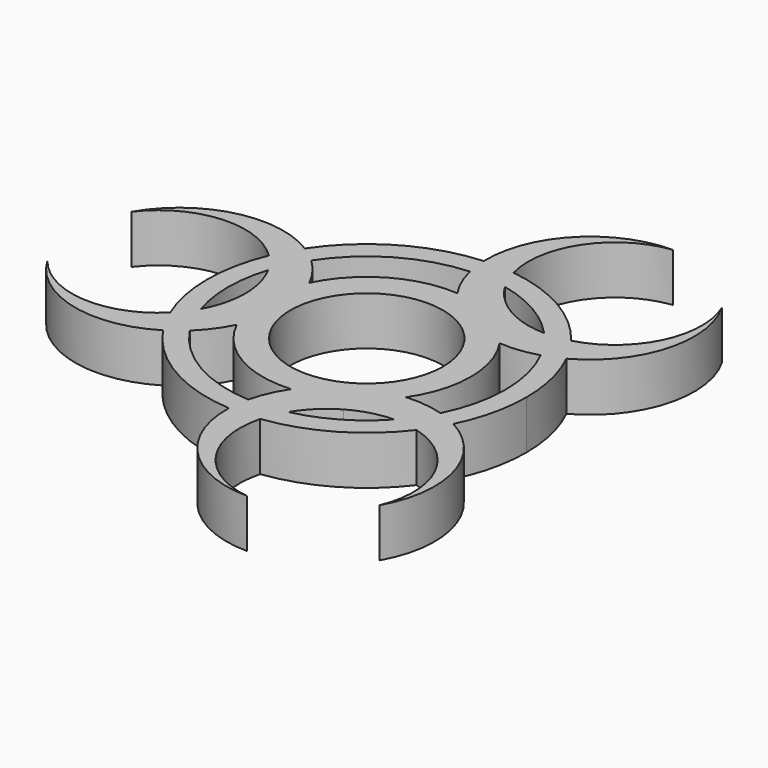
from build123d import *

# Parameters (mm, degrees)
F0_R     = 11
F1_DEPTH = 7
F2_COUNT = 3


# Not quite as in the source:
# - a feature names something its author has since deleted; it is built from what else it names


with BuildPart() as f1:
    # F0 (on Top) → F1 (new body)
    with BuildSketch(Plane.XY):
        with BuildLine():
            ThreePointArc((-13.5, -6.5383484153), (3.3541019662, -14.6201915172), (15, 0))
            ThreePointArc((15, 0), (3.3541019662, 14.6201915172), (-13.5, 6.5383484153))
            ThreePointArc((-13.5, 6.5383484153), (-12.3798084828, 3.3541019662), (-12, 0))
            ThreePointArc((-12, 0), (-12.3798084828, -3.3541019662), (-13.5, -6.5383484153))
        make_face()
        Circle(F0_R, mode=Mode.SUBTRACT)
        with BuildLine():
            ThreePointArc((-12, 0), (-12.3798084828, 3.3541019662), (-13.5, 6.5383484153))
            ThreePointArc((-13.5, 6.5383484153), (-15, 0), (-13.5, -6.5383484153))
            ThreePointArc((-13.5, -6.5383484153), (-12.3798084828, -3.3541019662), (-12, 0))
        make_face()
        with BuildLine():
            ThreePointArc((-13.5, -6.5383484153), (-15, 0), (-13.5, 6.5383484153))
            ThreePointArc((-13.5, 6.5383484153), (-14.9179607249, 8.8895628102), (-16.7407407407, 10.9429246297))
            ThreePointArc((-16.7407407407, 10.9429246297), (-18.0679116501, 8.5761628135), (-19.0625, 6.0515364784))
            ThreePointArc((-19.0625, 6.0515364784), (-17.8969270431, 3.125), (-17.5, 0))
            ThreePointArc((-17.5, 0), (-17.8969270431, -3.125), (-19.0625, -6.0515364784))
            ThreePointArc((-19.0625, -6.0515364784), (-18.0679116501, -8.5761628135), (-16.7407407407, -10.9429246297))
            ThreePointArc((-16.7407407407, -10.9429246297), (-14.9179607249, -8.8895628102), (-13.5, -6.5383484153))
        make_face()
        with BuildLine():
            ThreePointArc((-19.0625, 6.0515364784), (-18.0679116501, 8.5761628135), (-16.7407407407, 10.9429246297))
            ThreePointArc((-16.7407407407, 10.9429246297), (-17.8892997113, 11.9161713755), (-19.1296296296, 12.7693880133))
            ThreePointArc((-19.1296296296, 12.7693880133), (-20.264118899, 10.879590307), (-21.2125, 8.8898731009))
            ThreePointArc((-21.2125, 8.8898731009), (-20.0359172552, 7.5476522876), (-19.0625, 6.0515364784))
        make_face()
        with BuildLine():
            ThreePointArc((-19.1296296296, 12.7693880133), (-17.8892997113, 11.9161713755), (-16.7407407407, 10.9429246297))
            ThreePointArc((-16.7407407407, 10.9429246297), (5.7089922572, 19.1678743581), (20, 0))
            ThreePointArc((20, 0), (5.7089922572, -19.1678743581), (-16.7407407407, -10.9429246297))
            ThreePointArc((-16.7407407407, -10.9429246297), (-17.8892997113, -11.9161713755), (-19.1296296296, -12.7693880133))
            ThreePointArc((-19.1296296296, -12.7693880133), (6.6715260068, -22.011150373), (23, 0))
            ThreePointArc((23, 0), (6.6715260068, 22.011150373), (-19.1296296296, 12.7693880133))
        make_face()
        with BuildLine():
            ThreePointArc((-19.1296296296, -12.7693880133), (-17.8892997113, -11.9161713755), (-16.7407407407, -10.9429246297))
            ThreePointArc((-16.7407407407, -10.9429246297), (-18.0679116501, -8.5761628135), (-19.0625, -6.0515364784))
            ThreePointArc((-19.0625, -6.0515364784), (-20.0359172552, -7.5476522876), (-21.2125, -8.8898731009))
            ThreePointArc((-21.2125, -8.8898731009), (-20.264118899, -10.879590307), (-19.1296296296, -12.7693880133))
        make_face()
        with BuildLine():
            ThreePointArc((-21.2125, 8.8898731009), (-20.264118899, 10.879590307), (-19.1296296296, 12.7693880133))
            ThreePointArc((-19.1296296296, 12.7693880133), (-30.6426207614, 14.5509901377), (-39.9583333333, 7.5552364107))
            ThreePointArc((-39.9583333333, 7.5552364107), (-30.8877085374, 12.4684390985), (-21.2125, 8.8898731009))
        make_face()
        with BuildLine():
            ThreePointArc((-19.0625, -6.0515364784), (-20, 0), (-19.0625, 6.0515364784))
            ThreePointArc((-19.0625, 6.0515364784), (-20.0359172552, 7.5476522876), (-21.2125, 8.8898731009))
            ThreePointArc((-21.2125, 8.8898731009), (-23, 0), (-21.2125, -8.8898731009))
            ThreePointArc((-21.2125, -8.8898731009), (-20.0359172552, -7.5476522876), (-19.0625, -6.0515364784))
        make_face()
        with BuildLine():
            ThreePointArc((-39.9583333333, -7.5552364107), (-30.6426207614, -14.5509901377), (-19.1296296296, -12.7693880133))
            ThreePointArc((-19.1296296296, -12.7693880133), (-20.264118899, -10.879590307), (-21.2125, -8.8898731009))
            ThreePointArc((-21.2125, -8.8898731009), (-30.8877085374, -12.4684390985), (-39.9583333333, -7.5552364107))
        make_face()
    extrude(amount=F1_DEPTH)

    # F2: F1 ×3 about axis
    f2_axis = Axis((0, 0, 0), (0, 0, 1))


with BuildPart() as f1_1:
    add(f1.part)
    for i in range(1, F2_COUNT):
        add(f1.part.rotate(f2_axis, i * 360 / F2_COUNT))


solid = f1_1.part
